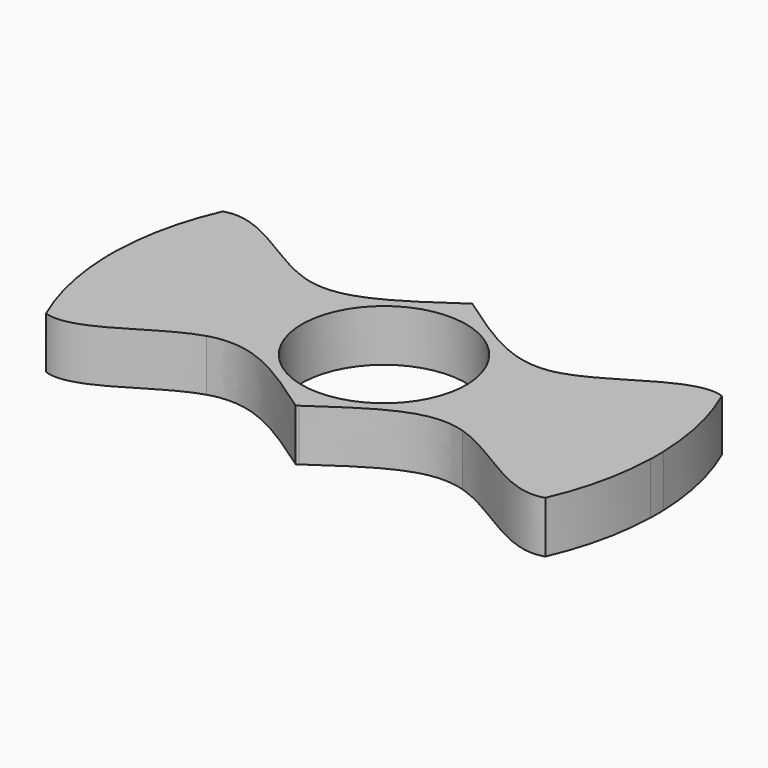
from build123d import *

# Parameters (mm, degrees)
F1_DEPTH = 7


with BuildPart() as f1:
    # F0 (on Top) → F1 (new body)
    with BuildSketch(Plane.XY):
        with BuildLine():
            ThreePointArc((0, 11.125), (7.8665629407, 7.8665629407), (11.125, 0))
            ThreePointArc((11.125, 0), (7.8665629407, -7.8665629407), (0, -11.125))
            Line((0, -11.125), (0, -14.935))
            add(Edge.make_bspline(
                [(0.2975305523, -14.7281560773), (0.1976224081, -14.7964212888), (0.098439929, -14.8653652618), (0, -14.935)],
                knots=[0.9970613329, 0.9970613329, 0.9970613329, 0.9970613329, 1, 1, 1, 1], degree=3))
            add(Edge.make_bspline(
                [(0.2975305523, -14.7281560773), (7.3951181082, -9.7951650898), (11.9191993362, -6.7662998847), (17.3106230519, -8.3854462868)],
                knots=[0.003112202, 0.003112202, 0.003112202, 0.003112202, 0.226966528, 0.226966528, 0.226966528, 0.226966528], degree=3))
            add(Edge.make_bspline(
                [(36.9228658424, -1.1001812607), (33.3191993332, -4.9864728132), (25.4350438971, -6.457479873), (17.3106230519, -8.3854462868)],
                knots=[0.6774767782, 0.6774767782, 0.6774767782, 0.6774767782, 0.8599164447, 0.8599164447, 0.8599164447, 0.8599164447], degree=3))
            ThreePointArc((36.9228658424, -1.1001812607), (36.9392531167, 0), (36.9228658424, 1.1001812607))
            add(Edge.make_bspline(
                [(36.9228658424, 1.1001812607), (33.3191993332, 4.9864728132), (25.4350438971, 6.457479873), (17.3106230519, 8.3854462868)],
                knots=[0.6774767782, 0.6774767782, 0.6774767782, 0.6774767782, 0.8599164447, 0.8599164447, 0.8599164447, 0.8599164447], degree=3))
            add(Edge.make_bspline(
                [(0.2975305523, 14.7281560773), (7.3951181082, 9.7951650898), (11.9191993362, 6.7662998847), (17.3106230519, 8.3854462868)],
                knots=[0.003112202, 0.003112202, 0.003112202, 0.003112202, 0.226966528, 0.226966528, 0.226966528, 0.226966528], degree=3))
            add(Edge.make_bspline(
                [(0.2975305523, 14.7281560773), (0.1976224081, 14.7964212888), (0.098439929, 14.8653652618), (0, 14.935)],
                knots=[0.9970613329, 0.9970613329, 0.9970613329, 0.9970613329, 1, 1, 1, 1], degree=3))
            Line((0, 14.935), (0, 11.125))
        make_face()
        with BuildLine():
            ThreePointArc((0, -11.125), (-11.125, 0), (0, 11.125))
            Line((0, 11.125), (0, 14.935))
            add(Edge.make_bspline(
                [(-0.2975305523, 14.7281560773), (-0.1976224081, 14.7964212888), (-0.098439929, 14.8653652618), (0, 14.935)],
                knots=[0.9970613329, 0.9970613329, 0.9970613329, 0.9970613329, 1, 1, 1, 1], degree=3))
            add(Edge.make_bspline(
                [(-0.2975305523, 14.7281560773), (-7.3951181082, 9.7951650898), (-11.9191993362, 6.7662998847), (-17.3106230519, 8.3854462868)],
                knots=[0.003112202, 0.003112202, 0.003112202, 0.003112202, 0.226966528, 0.226966528, 0.226966528, 0.226966528], degree=3))
            add(Edge.make_bspline(
                [(-36.9228658424, 1.1001812607), (-33.3191993332, 4.9864728132), (-25.4350438971, 6.457479873), (-17.3106230519, 8.3854462868)],
                knots=[0.6774767782, 0.6774767782, 0.6774767782, 0.6774767782, 0.8599164447, 0.8599164447, 0.8599164447, 0.8599164447], degree=3))
            ThreePointArc((-36.9228658424, 1.1001812607), (-36.9392531167, 0), (-36.9228658424, -1.1001812607))
            add(Edge.make_bspline(
                [(-36.9228658424, -1.1001812607), (-33.3191993332, -4.9864728132), (-25.4350438971, -6.457479873), (-17.3106230519, -8.3854462868)],
                knots=[0.6774767782, 0.6774767782, 0.6774767782, 0.6774767782, 0.8599164447, 0.8599164447, 0.8599164447, 0.8599164447], degree=3))
            add(Edge.make_bspline(
                [(-0.2975305523, -14.7281560773), (-7.3951181082, -9.7951650898), (-11.9191993362, -6.7662998847), (-17.3106230519, -8.3854462868)],
                knots=[0.003112202, 0.003112202, 0.003112202, 0.003112202, 0.226966528, 0.226966528, 0.226966528, 0.226966528], degree=3))
            add(Edge.make_bspline(
                [(-0.2975305523, -14.7281560773), (-0.1976224081, -14.7964212888), (-0.098439929, -14.8653652618), (0, -14.935)],
                knots=[0.9970613329, 0.9970613329, 0.9970613329, 0.9970613329, 1, 1, 1, 1], degree=3))
            Line((0, -14.935), (0, -11.125))
        make_face()
        with BuildLine():
            add(Edge.make_bspline(
                [(0, -14.935), (-0.0996804425, -14.865688897), (-0.1988542112, -14.796738465), (-0.2975305523, -14.7281560773)],
                knots=[0, 0, 0, 0, 0.003112202, 0.003112202, 0.003112202, 0.003112202], degree=3))
            add(Edge.make_bspline(
                [(-0.2975305523, -14.7281560773), (-0.1976224081, -14.7964212888), (-0.098439929, -14.8653652618), (0, -14.935)],
                knots=[0.9970613329, 0.9970613329, 0.9970613329, 0.9970613329, 1, 1, 1, 1], degree=3))
        make_face()
        with BuildLine():
            add(Edge.make_bspline(
                [(-36.9228658424, 1.1001812607), (-33.3191993332, 4.9864728132), (-25.4350438971, 6.457479873), (-17.3106230519, 8.3854462868)],
                knots=[0.6774767782, 0.6774767782, 0.6774767782, 0.6774767782, 0.8599164447, 0.8599164447, 0.8599164447, 0.8599164447], degree=3))
            add(Edge.make_bspline(
                [(-17.3106230519, 8.3854462868), (-17.3759482788, 8.4050646867), (-22.8109780057, 10.0907940795), (-29.1662144452, 16.5153198792), (-33.7854139507, 14.935)],
                knots=[0.226966528, 0.226966528, 0.226966528, 0.226966528, 0.2296788607, 0.4521923767, 0.4521923767, 0.4521923767, 0.4521923767], degree=3))
            ThreePointArc((-33.7854139507, 14.935), (-36.0245160996, 8.1696181434), (-36.9228658424, 1.1001812607))
        make_face()
        with BuildLine():
            add(Edge.make_bspline(
                [(17.3106230519, 8.3854462868), (17.3759482788, 8.4050646867), (22.8109780057, 10.0907940795), (29.1662144452, 16.5153198792), (33.7854139507, 14.935)],
                knots=[0.226966528, 0.226966528, 0.226966528, 0.226966528, 0.2296788607, 0.4521923767, 0.4521923767, 0.4521923767, 0.4521923767], degree=3))
            add(Edge.make_bspline(
                [(36.9228658424, 1.1001812607), (33.3191993332, 4.9864728132), (25.4350438971, 6.457479873), (17.3106230519, 8.3854462868)],
                knots=[0.6774767782, 0.6774767782, 0.6774767782, 0.6774767782, 0.8599164447, 0.8599164447, 0.8599164447, 0.8599164447], degree=3))
            ThreePointArc((36.9228658424, 1.1001812607), (36.0245160996, 8.1696181434), (33.7854139507, 14.935))
        make_face()
        with BuildLine():
            add(Edge.make_bspline(
                [(-17.3106230519, -8.3854462868), (-17.3759482788, -8.4050646867), (-22.8109780057, -10.0907940795), (-29.1662144452, -16.5153198792), (-33.7854139507, -14.935)],
                knots=[0.226966528, 0.226966528, 0.226966528, 0.226966528, 0.2296788607, 0.4521923767, 0.4521923767, 0.4521923767, 0.4521923767], degree=3))
            add(Edge.make_bspline(
                [(-36.9228658424, -1.1001812607), (-33.3191993332, -4.9864728132), (-25.4350438971, -6.457479873), (-17.3106230519, -8.3854462868)],
                knots=[0.6774767782, 0.6774767782, 0.6774767782, 0.6774767782, 0.8599164447, 0.8599164447, 0.8599164447, 0.8599164447], degree=3))
            ThreePointArc((-36.9228658424, -1.1001812607), (-36.0245160996, -8.1696181434), (-33.7854139507, -14.935))
        make_face()
        with BuildLine():
            add(Edge.make_bspline(
                [(36.9228658424, -1.1001812607), (33.3191993332, -4.9864728132), (25.4350438971, -6.457479873), (17.3106230519, -8.3854462868)],
                knots=[0.6774767782, 0.6774767782, 0.6774767782, 0.6774767782, 0.8599164447, 0.8599164447, 0.8599164447, 0.8599164447], degree=3))
            add(Edge.make_bspline(
                [(17.3106230519, -8.3854462868), (17.3759482788, -8.4050646867), (22.8109780057, -10.0907940795), (29.1662144452, -16.5153198792), (33.7854139507, -14.935)],
                knots=[0.226966528, 0.226966528, 0.226966528, 0.226966528, 0.2296788607, 0.4521923767, 0.4521923767, 0.4521923767, 0.4521923767], degree=3))
            ThreePointArc((33.7854139507, -14.935), (36.0245160996, -8.1696181434), (36.9228658424, -1.1001812607))
        make_face()
    extrude(amount=F1_DEPTH)


solid = f1.part
